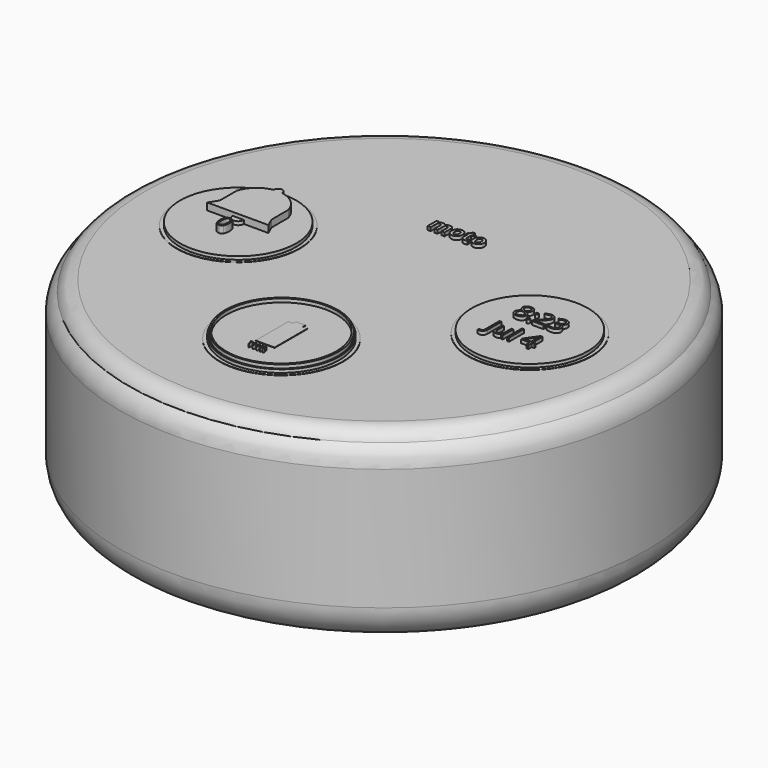
from build123d import *

# Parameters (mm, degrees)
F0_R          = 19.05
F1_DEPTH      = 12.7
F2_R          = 18.415
F3_DEPTH      = 0.762
F6_R          = 2.54
F7_R          = 3.5333997411
F7_R_2        = 1.6638979666
F8_DEPTH      = 0.0254
F9_DEPTH      = 0.0508
F10_R         = 4.191
F10_TEXT_SIZE = 1.4874780188
F11_DEPTH     = 0.254
F12_R         = 4.445
F13_DEPTH     = 0.0254
F15_DEPTH     = 0.0254
F16_DEPTH     = 0.0254
F17_DEPTH     = 0.254
F18_DEPTH     = 0.254
F21_TEXT_SIZE = 1.7774731128
F22_DEPTH     = 0.254
F23_W         = 3.7273742216
F23_H         = 1.524
F24_DEPTH     = 0.508
F25_DEPTH     = 0.254


# Not quite as in the source:
# - a fillet or chamfer that OpenCascade refuses, or shapes differently, is made with other operations: its cross-section is extruded or revolved along the edge and cut away or added
# - the program builds the solid bodies; features that only make, move or delete a surface that nothing else refers to are left out
# - Text() gives the source's letters only with a copy of the font that has no kerning and outlines rounded to 1/6400 em; it was checked with that copy


with BuildPart() as f1:
    # F0 (on Top) → F1 (new body)
    with BuildSketch(Plane.XY):
        Circle(F0_R)
    extrude(amount=F1_DEPTH)

    # F2 (on face) → F3 (join)
    with BuildSketch(Plane.XY.offset(12.7)):
        Circle(F2_R)
    extrude(amount=F3_DEPTH)

    # F4: fillet of radius 1.27 on 1 edges, made by hand

    # F4_s1 → F4_t2 (revolve, cut)
    with BuildSketch(Plane.XZ):
        with BuildLine():
            ThreePointArc((18.415, 12.7), (17.9466334215, 13.2545582337), (17.2510257735, 13.462))
            Line((17.2510257735, 13.462), (18.415, 13.462))
            Line((18.415, 13.462), (18.415, 12.7))
        make_face()
    revolve(axis=Axis((0, 0, 13.462), (0, 0, 1)), mode=Mode.SUBTRACT)

    # F5: fillet of radius 1.778 on 1 edges, made by hand

    # F5_s1 → F5_t2 (revolve, cut)
    with BuildSketch(Plane.XZ):
        with BuildLine():
            ThreePointArc((19.05, 11.3380767276), (18.8834493476, 12.08941886), (18.415, 12.7))
            Line((18.415, 12.7), (19.05, 12.7))
            Line((19.05, 12.7), (19.05, 11.3380767276))
        make_face()
    revolve(axis=Axis((0, 0, 12.7), (0, 0, 1)), mode=Mode.SUBTRACT)

    # F6
    f6_edges = [f1.edges().sort_by_distance(p)[0] for p in [
        (-19.05, 0, 0),
    ]]
    fillet(f6_edges, radius=F6_R)

    # F7 (on face) → F8 (join)
    with BuildSketch(Plane(origin=(0, 0, 0), x_dir=(1, 0, 0), z_dir=(0, 0, -1))):
        Circle(F7_R)
        Circle(F7_R_2, mode=Mode.SUBTRACT)
    extrude(amount=F8_DEPTH)

    # F9 (add): a face of the model
    f9_faces = [f1.faces().sort_by_distance(p)[0] for p in [
        (0, 0, 0),
    ]]
    extrude(f9_faces, amount=F9_DEPTH)

    # F10 (on face) → F11 (join)
    with BuildSketch(Plane.XY.offset(13.462)):
        with Locations((0, -9.2500257735)):
            Circle(F10_R)
        with Locations((10.5200257735, 0)):
            Circle(F10_R)
        with Locations((-10.5200257735, 0)):
            Circle(F10_R)
        with Locations((-1.9889208041, 6.2625310384)):
            Text('moto', F10_TEXT_SIZE, font='Open Sans', font_style=FontStyle.BOLD, text_align=(TextAlign.LEFT, TextAlign.BOTTOM))
    extrude(amount=F11_DEPTH)

    # F12 (on face) → F13 (join)
    with BuildSketch(Plane.XY.offset(13.462)):
        with Locations((-10.5200257735, 0)):
            Circle(F12_R)
        with Locations((0, -9.2500257735)):
            Circle(F12_R)
        with Locations((10.5200257735, 0)):
            Circle(F12_R)
    extrude(amount=F13_DEPTH)

    # F14 (on face) → F18 (join)
    with BuildSketch(Plane.XY.offset(13.716)):
        with BuildLine():
            add(Edge.make_bspline(
                [(0.0178840384, -11.3166332152), (-0.0003499051, -11.3517403603), (-0.0003499051, -11.4292637791)],
                knots=[0, 0, 0, 1, 1, 1], degree=2))
            add(Edge.make_bspline(
                [(-0.0003499051, -11.4292637791), (-0.0003499051, -11.5067871979), (0.0178840384, -11.5421664914)],
                knots=[0, 0, 0, 1, 1, 1], degree=2))
            add(Edge.make_bspline(
                [(0.0178840384, -11.5421664914), (0.036117982, -11.5775457849), (0.0759294067, -11.5775457849)],
                knots=[0, 0, 0, 1, 1, 1], degree=2))
            add(Edge.make_bspline(
                [(0.0759294067, -11.5775457849), (0.1162851283, -11.5775457849), (0.1343635584, -11.5416999513)],
                knots=[0, 0, 0, 1, 1, 1], degree=2))
            add(Edge.make_bspline(
                [(0.1343635584, -11.5416999513), (0.1524419886, -11.5058541177), (0.1524419886, -11.4292637791)],
                knots=[0, 0, 0, 1, 1, 1], degree=2))
            add(Edge.make_bspline(
                [(0.1524419886, -11.4292637791), (0.1524419886, -11.3527511972), (0.1343635584, -11.3171386337)],
                knots=[0, 0, 0, 1, 1, 1], degree=2))
            add(Edge.make_bspline(
                [(0.1343635584, -11.3171386337), (0.1162851283, -11.2815260702), (0.0759294067, -11.2815260702)],
                knots=[0, 0, 0, 1, 1, 1], degree=2))
            add(Edge.make_bspline(
                [(0.0759294067, -11.2815260702), (0.036117982, -11.2815260702), (0.0178840384, -11.3166332152)],
                knots=[0, 0, 0, 1, 1, 1], degree=2))
        make_face()
        with BuildLine():
            add(Edge.make_bspline(
                [(-0.2666276863, -11.3166332152), (-0.2848616298, -11.3517403603), (-0.2848616298, -11.4292637791)],
                knots=[0, 0, 0, 1, 1, 1], degree=2))
            add(Edge.make_bspline(
                [(-0.2848616298, -11.4292637791), (-0.2848616298, -11.5067871979), (-0.2666276863, -11.5421664914)],
                knots=[0, 0, 0, 1, 1, 1], degree=2))
            add(Edge.make_bspline(
                [(-0.2666276863, -11.5421664914), (-0.2483937427, -11.5775457849), (-0.208582318, -11.5775457849)],
                knots=[0, 0, 0, 1, 1, 1], degree=2))
            add(Edge.make_bspline(
                [(-0.208582318, -11.5775457849), (-0.1682265965, -11.5775457849), (-0.1501481663, -11.5416999513)],
                knots=[0, 0, 0, 1, 1, 1], degree=2))
            add(Edge.make_bspline(
                [(-0.1501481663, -11.5416999513), (-0.1320697361, -11.5058541177), (-0.1320697361, -11.4292637791)],
                knots=[0, 0, 0, 1, 1, 1], degree=2))
            add(Edge.make_bspline(
                [(-0.1320697361, -11.4292637791), (-0.1320697361, -11.3527511972), (-0.1501481663, -11.3171386337)],
                knots=[0, 0, 0, 1, 1, 1], degree=2))
            add(Edge.make_bspline(
                [(-0.1501481663, -11.3171386337), (-0.1682265965, -11.2815260702), (-0.208582318, -11.2815260702)],
                knots=[0, 0, 0, 1, 1, 1], degree=2))
            add(Edge.make_bspline(
                [(-0.208582318, -11.2815260702), (-0.2483937427, -11.2815260702), (-0.2666276863, -11.3166332152)],
                knots=[0, 0, 0, 1, 1, 1], degree=2))
        make_face()
        with BuildLine():
            Line((-0.5006364416, -11.6074043534), (-0.461291557, -11.6074043534))
            Line((-0.461291557, -11.6074043534), (-0.461291557, -11.2521340418))
            Line((-0.461291557, -11.2521340418), (-0.49527123, -11.2521340418))
            Line((-0.49527123, -11.2521340418), (-0.5892790669, -11.3248365459))
            Line((-0.5892790669, -11.3248365459), (-0.5678959775, -11.3525179271))
            add(Edge.make_bspline(
                [(-0.5100838793, -11.3051252252), (-0.5164210494, -11.3106848285), (-0.5678959775, -11.3525179271)],
                knots=[0, 0, 0, 1, 1, 1], degree=2))
            add(Edge.make_bspline(
                [(-0.4986925243, -11.2944336805), (-0.5037467091, -11.299565622), (-0.5100838793, -11.3051252252)],
                knots=[0, 0, 0, 1, 1, 1], degree=2))
            add(Edge.make_bspline(
                [(-0.5006364416, -11.3542285743), (-0.5006364416, -11.3225816019), (-0.4986925243, -11.2944336805)],
                knots=[0, 0, 0, 1, 1, 1], degree=2))
            Line((-0.5006364416, -11.3542285743), (-0.5006364416, -11.6074043534))
        make_face()
        with BuildLine():
            add(Edge.make_bspline(
                [(0.2863390069, -11.2963387194), (0.277319231, -11.3167498502), (0.277319231, -11.3581164087)],
                knots=[0, 0, 0, 1, 1, 1], degree=2))
            add(Edge.make_bspline(
                [(0.277319231, -11.3581164087), (0.277319231, -11.3994052106), (0.2863390069, -11.4200496115)],
                knots=[0, 0, 0, 1, 1, 1], degree=2))
            add(Edge.make_bspline(
                [(0.2863390069, -11.4200496115), (0.2953587828, -11.4406940124), (0.3154977653, -11.4406940124)],
                knots=[0, 0, 0, 1, 1, 1], degree=2))
            add(Edge.make_bspline(
                [(0.3154977653, -11.4406940124), (0.35530919, -11.4406940124), (0.35530919, -11.3581164087)],
                knots=[0, 0, 0, 1, 1, 1], degree=2))
            add(Edge.make_bspline(
                [(0.35530919, -11.3581164087), (0.35530919, -11.2759275886), (0.3154977653, -11.2759275886)],
                knots=[0, 0, 0, 1, 1, 1], degree=2))
            add(Edge.make_bspline(
                [(0.3154977653, -11.2759275886), (0.2953587828, -11.2759275886), (0.2863390069, -11.2963387194)],
                knots=[0, 0, 0, 1, 1, 1], degree=2))
        make_face()
        Polygon((0.3429458764, -11.6074043534), (0.5399813261, -11.2521340418), (0.5042910059, -11.2521340418), (0.3072555562, -11.6074043534), align=None)
        with BuildLine():
            add(Edge.make_bspline(
                [(0.5001699014, -11.4389056085), (0.4911501255, -11.4589668343), (0.4911501255, -11.5004889061)],
                knots=[0, 0, 0, 1, 1, 1], degree=2))
            add(Edge.make_bspline(
                [(0.4911501255, -11.5004889061), (0.4911501255, -11.542010978), (0.5001699014, -11.5625387439)],
                knots=[0, 0, 0, 1, 1, 1], degree=2))
            add(Edge.make_bspline(
                [(0.5001699014, -11.5625387439), (0.5091896773, -11.5830665098), (0.5295619298, -11.5830665098)],
                knots=[0, 0, 0, 1, 1, 1], degree=2))
            add(Edge.make_bspline(
                [(0.5295619298, -11.5830665098), (0.550011939, -11.5830665098), (0.5597315251, -11.5628108923)],
                knots=[0, 0, 0, 1, 1, 1], degree=2))
            add(Edge.make_bspline(
                [(0.5597315251, -11.5628108923), (0.5694511112, -11.5425552748), (0.5694511112, -11.5004889061)],
                knots=[0, 0, 0, 1, 1, 1], degree=2))
            add(Edge.make_bspline(
                [(0.5694511112, -11.5004889061), (0.5694511112, -11.4589668343), (0.5597315251, -11.4389056085)],
                knots=[0, 0, 0, 1, 1, 1], degree=2))
            add(Edge.make_bspline(
                [(0.5597315251, -11.4389056085), (0.550011939, -11.4188443828), (0.5295619298, -11.4188443828)],
                knots=[0, 0, 0, 1, 1, 1], degree=2))
            add(Edge.make_bspline(
                [(0.5295619298, -11.4188443828), (0.5091896773, -11.4188443828), (0.5001699014, -11.4389056085)],
                knots=[0, 0, 0, 1, 1, 1], degree=2))
        make_face()
    extrude(amount=F18_DEPTH)


with BuildPart() as f15:
    # F14 (on face) → F15 (new body)
    with BuildSketch(Plane.XY.offset(13.716)):
        Polygon((-0.6859390996, -7.7759823762), (-0.6859390996, -10.7240691708), (0.6859390996, -10.7240691708), (0.6859390996, -7.7759823762), (0.3471470554, -7.7759823762), (0.3471470554, -7.5169056654), (-0.3471470554, -7.5169056654), (-0.3471470554, -7.7759823762), align=None)
    extrude(amount=F15_DEPTH)


with BuildPart() as f16:
    # F14 (on face) → F16 (new body)
    with BuildSketch(Plane.XY.offset(13.716)):
        with BuildLine():
            ThreePointArc((0, -5.1606257735), (-4.0795815144, -9.2500257735), (0, -13.3394257735))
            ThreePointArc((0, -13.3394257735), (4.0894, -9.2500257735), (0, -5.1606257735))
        make_face()
        with BuildLine():
            ThreePointArc((0, -5.2622257735), (3.9585404882, -9.2500257735), (0, -13.2378257735))
            ThreePointArc((0, -13.2378257735), (-3.9617719224, -9.2500257735), (0, -5.2622257735))
        make_face(mode=Mode.SUBTRACT)
    extrude(amount=F16_DEPTH)


with BuildPart() as f17:
    # F14 (on face) → F17 (new body)
    with BuildSketch(Plane.XY.offset(13.716)):
        with BuildLine():
            ThreePointArc((0, -5.1606257735), (-4.0795815144, -9.2500257735), (0, -13.3394257735))
            ThreePointArc((0, -13.3394257735), (4.0894, -9.2500257735), (0, -5.1606257735))
        make_face()
        with BuildLine():
            ThreePointArc((0, -5.2622257735), (3.9585404882, -9.2500257735), (0, -13.2378257735))
            ThreePointArc((0, -13.2378257735), (-3.9617719224, -9.2500257735), (0, -5.2622257735))
        make_face(mode=Mode.SUBTRACT)
    extrude(amount=F17_DEPTH)


with BuildPart() as f22:
    # F21 (on face) → F22 (new body)
    with BuildSketch(Plane.XY.offset(13.716)):
        with Locations((8.6640938866, 0.5213923578)):
            Text('8:23', F21_TEXT_SIZE, font='Open Sans', text_align=(TextAlign.LEFT, TextAlign.BOTTOM))
        with Locations((8.6640938866, -1.8959710756)):
            Text('Jul 4', F21_TEXT_SIZE, font='Open Sans', text_align=(TextAlign.LEFT, TextAlign.BOTTOM))
    extrude(amount=F22_DEPTH)


with BuildPart() as f24:
    # F23 (on face) → F24 (new body)
    with BuildSketch(Plane.XY.offset(13.716)):
        Polygon((-10.9330574051, 0), (-10.5200257735, 0), (-10.1069941419, 0), (-8.3463426947, 0), (-8.621764018, 0.6281484183), (-12.3491382397, 0.6281484183), (-12.75308999, 0), align=None)
        with Locations((-10.4854511289, 1.3901484183)):
            Rectangle(F23_W, F23_H)
        with BuildLine():
            ThreePointArc((-10.7955552317, 3.5305359685), (-11.7724360238, 3.0668631784), (-12.3491382397, 2.1521484183))
            Line((-12.3491382397, 2.1521484183), (-8.621764018, 2.1521484183))
            ThreePointArc((-8.621764018, 2.1521484183), (-9.1984662339, 3.0668631784), (-10.175347026, 3.5305359685))
            ThreePointArc((-10.175347026, 3.5305359685), (-10.4854511289, 3.5554915611), (-10.7955552317, 3.5305359685))
        make_face()
        with BuildLine():
            ThreePointArc((-10.175347026, 3.5305359685), (-10.4854511289, 3.8665981927), (-10.7955552317, 3.5305359685))
            ThreePointArc((-10.7955552317, 3.5305359685), (-10.4854511289, 3.5554915611), (-10.175347026, 3.5305359685))
        make_face()
    extrude(amount=F24_DEPTH)


with BuildPart() as f24b:
    # F23 (on face) → F24, piece 2 (new body)
    with BuildSketch(Plane.XY.offset(13.716)):
        with BuildLine():
            Line((-10.5200257735, -0.7868447211), (-10.5200257735, -0.6861075819))
            add(Edge.make_bspline(
                [(-10.53187852, -0.6859333582), (-10.5259004714, -0.6859333582), (-10.5200257735, -0.6861075819)],
                knots=[0, 0, 0, 0.0359288548, 0.0359288548, 0.0359288548], degree=2))
            add(Edge.make_bspline(
                [(-10.7854825671, -0.8153072042), (-10.7022897051, -0.6859333582), (-10.53187852, -0.6859333582)],
                knots=[0, 0, 0, 1, 1, 1], degree=2))
            add(Edge.make_bspline(
                [(-10.8686754291, -1.2114796641), (-10.8686754291, -0.9446810501), (-10.7854825671, -0.8153072042)],
                knots=[0, 0, 0, 1, 1, 1], degree=2))
            add(Edge.make_bspline(
                [(-10.782687108, -1.6040739364), (-10.8686754291, -1.4702273559), (-10.8686754291, -1.2114796641)],
                knots=[0, 0, 0, 1, 1, 1], degree=2))
            add(Edge.make_bspline(
                [(-10.53187852, -1.7379205168), (-10.6966987869, -1.7379205168), (-10.782687108, -1.6040739364)],
                knots=[0, 0, 0, 1, 1, 1], degree=2))
            add(Edge.make_bspline(
                [(-10.5200257735, -1.7377624764), (-10.525898678, -1.7379205168), (-10.53187852, -1.7379205168)],
                knots=[0.9652287548, 0.9652287548, 0.9652287548, 1, 1, 1], degree=2))
            Line((-10.5200257735, -1.7377624764), (-10.5200257735, -1.6376782639))
            add(Edge.make_bspline(
                [(-10.53187852, -1.6379549003), (-10.5258661854, -1.6379549003), (-10.5200257735, -1.6376782639)],
                knots=[0, 0, 0, 0.0518003454, 0.0518003454, 0.0518003454], degree=2))
            add(Edge.make_bspline(
                [(-10.6988233358, -1.53620019), (-10.6463805236, -1.6379549003), (-10.53187852, -1.6379549003)],
                knots=[0, 0, 0, 1, 1, 1], degree=2))
            add(Edge.make_bspline(
                [(-10.751266148, -1.2114796641), (-10.751266148, -1.4344454798), (-10.6988233358, -1.53620019)],
                knots=[0, 0, 0, 1, 1, 1], degree=2))
            add(Edge.make_bspline(
                [(-10.6988233358, -0.8875418666), (-10.751266148, -0.9885138484), (-10.751266148, -1.2114796641)],
                knots=[0, 0, 0, 1, 1, 1], degree=2))
            add(Edge.make_bspline(
                [(-10.53187852, -0.7865698849), (-10.6463805236, -0.7865698849), (-10.6988233358, -0.8875418666)],
                knots=[0, 0, 0, 1, 1, 1], degree=2))
            add(Edge.make_bspline(
                [(-10.5200257735, -0.7868447211), (-10.5258661854, -0.7865698849), (-10.53187852, -0.7865698849)],
                knots=[0.9481996546, 0.9481996546, 0.9481996546, 1, 1, 1], degree=2))
        make_face()
        with BuildLine():
            add(Edge.make_bspline(
                [(-10.5200257735, -0.6861075819), (-10.3623912815, -0.6907824876), (-10.2791690197, -0.8208981223)],
                knots=[0.0359288548, 0.0359288548, 0.0359288548, 1, 1, 1], degree=2))
            Line((-10.5200257735, -0.6861075819), (-10.5200257735, -0.7868447211))
            add(Edge.make_bspline(
                [(-10.3638155204, -0.8889955053), (-10.4131176724, -0.7918755674), (-10.5200257735, -0.7868447211)],
                knots=[0, 0, 0, 0.9481996546, 0.9481996546, 0.9481996546], degree=2))
            add(Edge.make_bspline(
                [(-10.3118199817, -1.2114796641), (-10.3118199817, -0.9914211258), (-10.3638155204, -0.8889955053)],
                knots=[0, 0, 0, 1, 1, 1], degree=2))
            add(Edge.make_bspline(
                [(-10.3638155204, -1.5348583697), (-10.3118199817, -1.4317618391), (-10.3118199817, -1.2114796641)],
                knots=[0, 0, 0, 1, 1, 1], degree=2))
            add(Edge.make_bspline(
                [(-10.5200257735, -1.6376782639), (-10.4131176724, -1.6326144644), (-10.3638155204, -1.5348583697)],
                knots=[0.0518003454, 0.0518003454, 0.0518003454, 1, 1, 1], degree=2))
            Line((-10.5200257735, -1.6376782639), (-10.5200257735, -1.7377624764))
            add(Edge.make_bspline(
                [(-10.2763735606, -1.6072048505), (-10.3569974941, -1.7333753703), (-10.5200257735, -1.7377624764)],
                knots=[0, 0, 0, 0.9652287548, 0.9652287548, 0.9652287548], degree=2))
            add(Edge.make_bspline(
                [(-10.1928452435, -1.2114796641), (-10.1928452435, -1.4764891842), (-10.2763735606, -1.6072048505)],
                knots=[0, 0, 0, 1, 1, 1], degree=2))
            add(Edge.make_bspline(
                [(-10.2791690197, -0.8208981223), (-10.1928452435, -0.9558628864), (-10.1928452435, -1.2114796641)],
                knots=[0, 0, 0, 1, 1, 1], degree=2))
        make_face()
    extrude(amount=F24_DEPTH)


with BuildPart() as f25:
    # F23 (on face) → F25 (new body)
    with BuildSketch(Plane.XY.offset(13.716)):
        with BuildLine():
            Line((-10.5200257735, -0.4130316316), (-10.5200257735, 0))
            Line((-10.5200257735, 0), (-10.9330574051, 0))
            ThreePointArc((-10.9330574051, 0), (-10.812083241, -0.2920574675), (-10.5200257735, -0.4130316316))
        make_face()
        with BuildLine():
            Line((-10.1069941419, 0), (-10.5200257735, 0))
            Line((-10.5200257735, 0), (-10.5200257735, -0.4130316316))
            ThreePointArc((-10.5200257735, -0.4130316316), (-10.227968306, -0.2920574675), (-10.1069941419, 0))
        make_face()
    extrude(amount=F25_DEPTH)


solid = Compound([f1.part, f15.part, f16.part, f17.part, f22.part, f24.part, f24b.part, f25.part])
